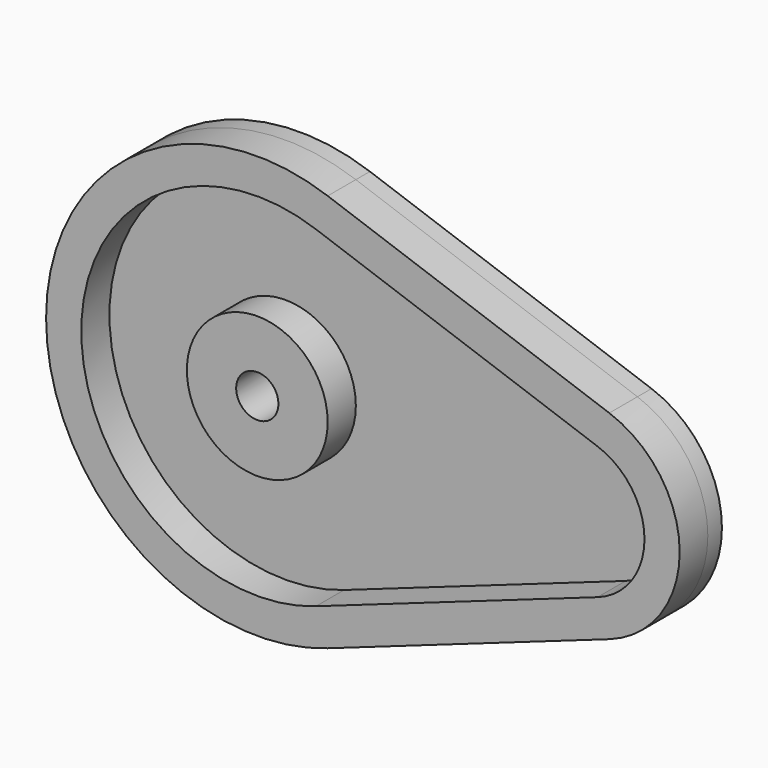
from build123d import *
from build123d import SkipClean  # not in build123d's __all__

# Parameters (mm, degrees)
F1_DEPTH = 10
F0_R     = 20
F3_DEPTH = 5
F5_D     = 12
F5_DEPTH = 15
F5_TIP   = 3.6051637142


# Not quite as in the source:
# - after a boolean that leaves OpenCascade's solid faulty, fix() repairs it


with BuildPart() as f1:
    # F0 (on Front) → F1 (new body)
    with BuildSketch(Plane.XZ):
        with BuildLine():
            Line((10, 28.2842712475), (-70, 56.5685424949))
            ThreePointArc((-70, 56.5685424949), (-150, 0), (-70, -56.5685424949))
            Line((-70, -56.5685424949), (10, -28.2842712475))
            ThreePointArc((10, -28.2842712475), (30, 0), (10, 28.2842712475))
        make_face()
        with BuildLine():
            ThreePointArc((-73.3333333333, -47.1404520791), (-140, 0), (-73.3333333333, 47.1404520791))
            Line((-73.3333333333, 47.1404520791), (6.6666666667, 18.8561808316))
            ThreePointArc((6.6666666667, 18.8561808316), (20, 0), (6.6666666667, -18.8561808316))
            Line((6.6666666667, -18.8561808316), (-73.3333333333, -47.1404520791))
        make_face(mode=Mode.SUBTRACT)
    extrude(amount=F1_DEPTH)



with BuildPart() as f1b:
    # F0 (on Front) → F1, piece 2 (new body)
    with BuildSketch(Plane.XZ):
        with Locations((-90, 0)):
            Circle(F0_R)
    extrude(amount=F1_DEPTH)


with BuildPart() as f1_1:
    add(f1.part, clean=False)

    with SkipClean():  # cleaning this boolean's faces spoils the solid; the shape is the same uncleaned
        add(f1b.part)  # F3 merges F1b
    # F2 (on face) → F3 (join)
    with BuildSketch(Plane(origin=(0, 0, 0), x_dir=(-1, 0, 0), z_dir=(0, 1, 0))):
        with BuildLine():
            ThreePointArc((70, -56.5685424949), (150, 0), (70, 56.5685424949))
            Line((70, 56.5685424949), (-10, 28.2842712475))
            ThreePointArc((-10, 28.2842712475), (-30, 0), (-10, -28.2842712475))
            Line((-10, -28.2842712475), (70, -56.5685424949))
        make_face()
    with SkipClean():  # cleaning this boolean's faces spoils the solid; the shape is the same uncleaned
        extrude(amount=F3_DEPTH)

    # F5
    with Locations(Plane.XZ.offset(10)):
        with Locations((-90, 0)):
            Hole(F5_D / 2, depth=F5_DEPTH)
            with Locations((0, 0, -(F5_DEPTH + F5_TIP / 2))):  # 118° drill point
                Cone(0, F5_D / 2, F5_TIP, mode=Mode.SUBTRACT)

    add(f1_1.part.fix(), mode=Mode.REPLACE)


solid = f1_1.part
